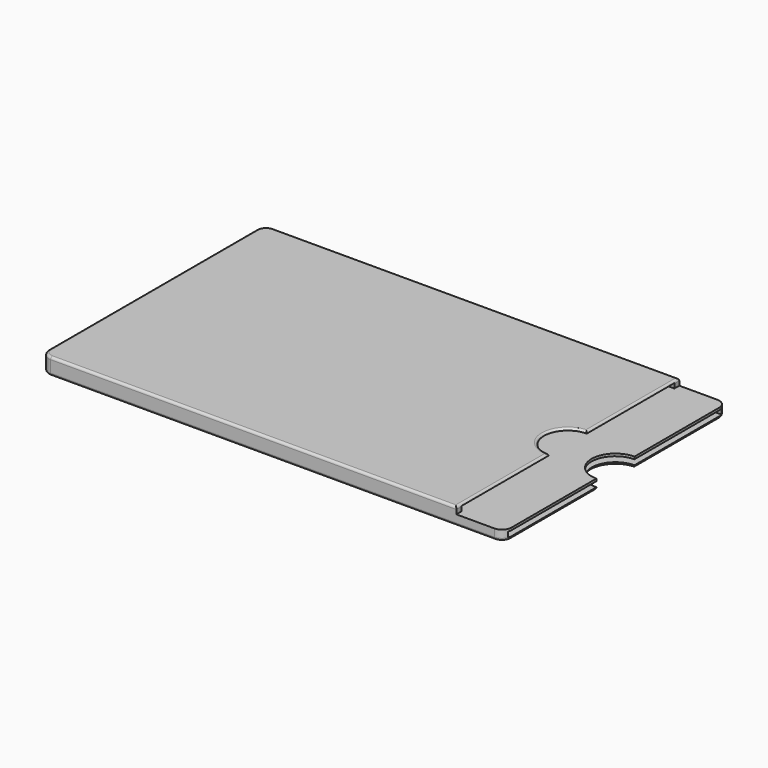
from build123d import *

# Parameters (mm, degrees)
F0_W         = 10
F0_H         = 56
F1_DEPTH     = 3
F2_DEPTH     = 2.6
F4_DEPTH     = 1.6
F5_DEPTH     = 1.1
F6_DEPTH     = 0.5
F7_T1_DEPTH  = 13.5
F7_T3_DEPTH  = 12.1
F8_T1_DEPTH  = 86.55
F8_T3_DEPTH  = 54.6
F8_T5_DEPTH  = 26.8
F8_T7_DEPTH  = 26.8
F8_T9_DEPTH  = 93.3
F8_T11_DEPTH = 23.55
F8_T13_DEPTH = 23.55
F8_T16_ANGLE = 89.9999999857
F8_T18_ANGLE = 208.1142252403
F8_T20_ANGLE = 89.9999999955
F8_T22_ANGLE = 89.9999999857
F8_T24_ANGLE = 89.9999999955
F8_T26_ANGLE = 208.6939609801
F8_T28_ANGLE = 90.0000000053
F8_T30_ANGLE = 89.9999999955


# Not quite as in the source:
# - a fillet or chamfer that OpenCascade refuses, or shapes differently, is made with other operations: its cross-section is extruded or revolved along the edge and cut away or added


with BuildPart() as f1:
    # F0 (on Top) → F1 (new body)
    with BuildSketch(Plane.XY):
        Polygon((-58.3780704141, -12.1535575017), (-58.3780704141, 43.8464424983), (-48.3780704141, 43.8464424983), (27.6219295859, 43.8464424983), (27.6219295859, 45.1464424983), (-59.6780704141, 45.1464424983), (-59.6780704141, -13.4535575017), (27.6219295859, -13.4535575017), (27.6219295859, -12.1535575017), (-48.3780704141, -12.1535575017), align=None)
        with Locations((-53.3780704141, 15.8464424983)):
            Rectangle(F0_W, F0_H)
        with BuildLine():
            Line((27.6219295859, 43.8464424983), (-48.3780704141, 43.8464424983))
            Line((-48.3780704141, 43.8464424983), (-48.3780704141, -12.1535575017))
            Line((-48.3780704141, -12.1535575017), (27.6219295859, -12.1535575017))
            Line((27.6219295859, -12.1535575017), (27.6219295859, 10.8464424983))
            ThreePointArc((27.6219295859, 10.8464424983), (22.6219295859, 15.8464424983), (27.6219295859, 20.8464424983))
            Line((27.6219295859, 20.8464424983), (27.6219295859, 43.8464424983))
        make_face()
    extrude(amount=F1_DEPTH)

    # F0 (on Top) → F2 (cut)
    with BuildSketch(Plane.XY):
        with Locations((-53.3780704141, 15.8464424983)):
            Rectangle(F0_W, F0_H)
        with BuildLine():
            Line((27.6219295859, 43.8464424983), (-48.3780704141, 43.8464424983))
            Line((-48.3780704141, 43.8464424983), (-48.3780704141, -12.1535575017))
            Line((-48.3780704141, -12.1535575017), (27.6219295859, -12.1535575017))
            Line((27.6219295859, -12.1535575017), (27.6219295859, 10.8464424983))
            ThreePointArc((27.6219295859, 10.8464424983), (22.6219295859, 15.8464424983), (27.6219295859, 20.8464424983))
            Line((27.6219295859, 20.8464424983), (27.6219295859, 43.8464424983))
        make_face()
    extrude(amount=F2_DEPTH, mode=Mode.SUBTRACT)

    # F0 (on Top) + F3 (on Top) → F4 (join)
    with BuildSketch(Plane.XY):
        with BuildLine():
            Line((27.6219295859, 43.8464424983), (-48.3780704141, 43.8464424983))
            Line((-48.3780704141, 43.8464424983), (-48.3780704141, -12.1535575017))
            Line((-48.3780704141, -12.1535575017), (27.6219295859, -12.1535575017))
            Line((27.6219295859, -12.1535575017), (27.6219295859, 10.8464424983))
            ThreePointArc((27.6219295859, 10.8464424983), (22.6219295859, 15.8464424983), (27.6219295859, 20.8464424983))
            Line((27.6219295859, 20.8464424983), (27.6219295859, 43.8464424983))
        make_face()
        with BuildLine():
            Line((27.6219295859, 10.8464424983), (27.6219295859, 20.8464424983))
            ThreePointArc((27.6219295859, 20.8464424983), (22.6219295859, 15.8464424983), (27.6219295859, 10.8464424983))
        make_face()
        with Locations((-53.3780704141, 15.8464424983)):
            Rectangle(F0_W, F0_H)
    with BuildSketch(Plane.XY):
        with BuildLine():
            Line((37.6219295859, 20.8464424983), (37.6219295859, 45.1464424983))
            Line((37.6219295859, 45.1464424983), (27.6219295859, 45.1464424983))
            Line((27.6219295859, 45.1464424983), (27.6219295859, -13.4535575017))
            Line((27.6219295859, -13.4535575017), (37.6219295859, -13.4535575017))
            Line((37.6219295859, -13.4535575017), (37.6219295859, 10.8464424983))
            ThreePointArc((37.6219295859, 10.8464424983), (32.6219295859, 15.8464424983), (37.6219295859, 20.8464424983))
        make_face()
    extrude(amount=F4_DEPTH)

    # F0 (on Top) → F5 (cut)
    with BuildSketch(Plane.XY):
        Polygon((37.6219295859, 43.8464424983), (27.6219295859, 43.8464424983), (27.6219295859, 20.8464424983), (27.6219295859, 10.8464424983), (27.6219295859, -12.1535575017), (37.6219295859, -12.1535575017), align=None)
        with BuildLine():
            Line((27.6219295859, 43.8464424983), (-48.3780704141, 43.8464424983))
            Line((-48.3780704141, 43.8464424983), (-48.3780704141, -12.1535575017))
            Line((-48.3780704141, -12.1535575017), (27.6219295859, -12.1535575017))
            Line((27.6219295859, -12.1535575017), (27.6219295859, 10.8464424983))
            ThreePointArc((27.6219295859, 10.8464424983), (22.6219295859, 15.8464424983), (27.6219295859, 20.8464424983))
            Line((27.6219295859, 20.8464424983), (27.6219295859, 43.8464424983))
        make_face()
        with BuildLine():
            Line((27.6219295859, 10.8464424983), (27.6219295859, 20.8464424983))
            ThreePointArc((27.6219295859, 20.8464424983), (22.6219295859, 15.8464424983), (27.6219295859, 10.8464424983))
        make_face()
    extrude(amount=F5_DEPTH, mode=Mode.SUBTRACT)

    # F0 (on Top) + F3 (on Top) → F6 (join)
    with BuildSketch(Plane.XY):
        with BuildLine():
            Line((27.6219295859, 43.8464424983), (-48.3780704141, 43.8464424983))
            Line((-48.3780704141, 43.8464424983), (-48.3780704141, -12.1535575017))
            Line((-48.3780704141, -12.1535575017), (27.6219295859, -12.1535575017))
            Line((27.6219295859, -12.1535575017), (27.6219295859, 10.8464424983))
            ThreePointArc((27.6219295859, 10.8464424983), (22.6219295859, 15.8464424983), (27.6219295859, 20.8464424983))
            Line((27.6219295859, 20.8464424983), (27.6219295859, 43.8464424983))
        make_face()
        with BuildLine():
            Line((27.6219295859, 10.8464424983), (27.6219295859, 20.8464424983))
            ThreePointArc((27.6219295859, 20.8464424983), (22.6219295859, 15.8464424983), (27.6219295859, 10.8464424983))
        make_face()
        with Locations((-53.3780704141, 15.8464424983)):
            Rectangle(F0_W, F0_H)
        Polygon((-58.3780704141, -12.1535575017), (-58.3780704141, 43.8464424983), (-48.3780704141, 43.8464424983), (27.6219295859, 43.8464424983), (27.6219295859, 45.1464424983), (-59.6780704141, 45.1464424983), (-59.6780704141, -13.4535575017), (27.6219295859, -13.4535575017), (27.6219295859, -12.1535575017), (-48.3780704141, -12.1535575017), align=None)
    with BuildSketch(Plane.XY):
        with BuildLine():
            Line((37.6219295859, 20.8464424983), (37.6219295859, 45.1464424983))
            Line((37.6219295859, 45.1464424983), (27.6219295859, 45.1464424983))
            Line((27.6219295859, 45.1464424983), (27.6219295859, -13.4535575017))
            Line((27.6219295859, -13.4535575017), (37.6219295859, -13.4535575017))
            Line((37.6219295859, -13.4535575017), (37.6219295859, 10.8464424983))
            ThreePointArc((37.6219295859, 10.8464424983), (32.6219295859, 15.8464424983), (37.6219295859, 20.8464424983))
        make_face()
    extrude(amount=-F6_DEPTH)

    # F7: fillet of radius 2 on 4 edges, made by hand

    # F7_s2 → F7_t1 (cut)
    with BuildSketch(Plane.XY.offset(-5.5)):
        with BuildLine():
            ThreePointArc((-57.6780704141, 45.1464424983), (-59.0922839764, 44.5606560606), (-59.6780704141, 43.1464424983))
            Line((-59.6780704141, 43.1464424983), (-59.6780704141, 45.1464424983))
            Line((-59.6780704141, 45.1464424983), (-57.6780704141, 45.1464424983))
        make_face()
        with BuildLine():
            ThreePointArc((-57.6780704141, -13.4535575017), (-59.0922839764, -12.8677710641), (-59.6780704141, -11.4535575017))
            Line((-59.6780704141, -11.4535575017), (-59.6780704141, -13.4535575017))
            Line((-59.6780704141, -13.4535575017), (-57.6780704141, -13.4535575017))
        make_face()
    extrude(amount=F7_T1_DEPTH, mode=Mode.SUBTRACT)

    # F7_s4 → F7_t3 (cut)
    with BuildSketch(Plane.XY.offset(-5.5)):
        with BuildLine():
            ThreePointArc((37.6219295859, -11.4535575017), (37.0361431483, -12.8677710641), (35.6219295859, -13.4535575017))
            Line((35.6219295859, -13.4535575017), (37.6219295859, -13.4535575017))
            Line((37.6219295859, -13.4535575017), (37.6219295859, -11.4535575017))
        make_face()
        with BuildLine():
            ThreePointArc((35.6219295859, 45.1464424983), (37.0361431483, 44.5606560606), (37.6219295859, 43.1464424983))
            Line((37.6219295859, 43.1464424983), (37.6219295859, 45.1464424983))
            Line((37.6219295859, 45.1464424983), (35.6219295859, 45.1464424983))
        make_face()
    extrude(amount=F7_T3_DEPTH, mode=Mode.SUBTRACT)

    # F8: fillet of radius 0.5 on 18 edges, made by hand

    # F8_s2 → F8_t1 (cut)
    with BuildSketch(Plane.YZ.offset(-57.6780704141)):
        with BuildLine():
            ThreePointArc((45.1464424983, 2.5), (44.9999958889, 2.8535533906), (44.6464424983, 3))
            Line((44.6464424983, 3), (45.1464424983, 3))
            Line((45.1464424983, 3), (45.1464424983, 2.5))
        make_face()
        with BuildLine():
            ThreePointArc((-12.9535575017, 3), (-13.3071108923, 2.8535533906), (-13.4535575017, 2.5))
            Line((-13.4535575017, 2.5), (-13.4535575017, 3))
            Line((-13.4535575017, 3), (-12.9535575017, 3))
        make_face()
    extrude(amount=F8_T1_DEPTH, mode=Mode.SUBTRACT)

    # F8_s4 → F8_t3 (cut)
    with BuildSketch(Plane.XZ.offset(-43.1464424983)):
        with BuildLine():
            ThreePointArc((-59.1780704141, 3), (-59.5316238047, 2.8535533906), (-59.6780704141, 2.5))
            Line((-59.6780704141, 2.5), (-59.6780704141, 3))
            Line((-59.6780704141, 3), (-59.1780704141, 3))
        make_face()
        with BuildLine():
            ThreePointArc((-59.1780704141, -0.5), (-59.5316238047, -0.3535533906), (-59.6780704141, 0))
            Line((-59.6780704141, 0), (-59.6780704141, -0.5))
            Line((-59.6780704141, -0.5), (-59.1780704141, -0.5))
        make_face()
    extrude(amount=F8_T3_DEPTH, mode=Mode.SUBTRACT)

    # F8_s6 → F8_t5 (cut)
    with BuildSketch(Plane.XZ.offset(-46.3964424983)):
        with BuildLine():
            ThreePointArc((27.1219295859, 3), (27.4754829765, 2.8535533906), (27.6219295859, 2.5))
            Line((27.6219295859, 2.5), (27.6219295859, 3))
            Line((27.6219295859, 3), (27.1219295859, 3))
        make_face()
    extrude(amount=F8_T5_DEPTH, mode=Mode.SUBTRACT)

    # F8_s8 → F8_t7 (cut)
    with BuildSketch(Plane.XZ.offset(-12.0964424983)):
        with BuildLine():
            ThreePointArc((27.1219295859, 3), (27.4754829765, 2.8535533906), (27.6219295859, 2.5))
            Line((27.6219295859, 2.5), (27.6219295859, 3))
            Line((27.6219295859, 3), (27.1219295859, 3))
        make_face()
    extrude(amount=F8_T7_DEPTH, mode=Mode.SUBTRACT)

    # F8_s10 → F8_t9 (cut)
    with BuildSketch(Plane.YZ.offset(-57.6780704141)):
        with BuildLine():
            ThreePointArc((45.1464424983, 0), (44.9999958889, -0.3535533906), (44.6464424983, -0.5))
            Line((44.6464424983, -0.5), (45.1464424983, -0.5))
            Line((45.1464424983, -0.5), (45.1464424983, 0))
        make_face()
        with BuildLine():
            ThreePointArc((-12.9535575017, -0.5), (-13.3071108923, -0.3535533906), (-13.4535575017, 0))
            Line((-13.4535575017, 0), (-13.4535575017, -0.5))
            Line((-13.4535575017, -0.5), (-12.9535575017, -0.5))
        make_face()
    extrude(amount=F8_T9_DEPTH, mode=Mode.SUBTRACT)

    # F8_s12 → F8_t11 (cut)
    with BuildSketch(Plane.XZ.offset(-43.1464424983)):
        with BuildLine():
            ThreePointArc((37.1219295859, -0.5), (37.4754829765, -0.3535533906), (37.6219295859, 0))
            Line((37.6219295859, 0), (37.6219295859, -0.5))
            Line((37.6219295859, -0.5), (37.1219295859, -0.5))
        make_face()
    extrude(amount=F8_T11_DEPTH, mode=Mode.SUBTRACT)

    # F8_s14 → F8_t13 (cut)
    with BuildSketch(Plane.XZ.offset(-12.0964424983)):
        with BuildLine():
            ThreePointArc((37.1219295859, -0.5), (37.4754829765, -0.3535533906), (37.6219295859, 0))
            Line((37.6219295859, 0), (37.6219295859, -0.5))
            Line((37.6219295859, -0.5), (37.1219295859, -0.5))
        make_face()
    extrude(amount=F8_T13_DEPTH, mode=Mode.SUBTRACT)

    # F8_s15 → F8_t16 (revolve, cut)
    with BuildSketch(Plane.XZ.offset(-43.1464424981)):
        with BuildLine():
            ThreePointArc((-59.6780704141, 2.5), (-59.5316238047, 2.8535533906), (-59.1780704141, 3))
            Line((-59.1780704141, 3), (-59.6780704141, 3))
            Line((-59.6780704141, 3), (-59.6780704141, 2.5))
        make_face()
    revolve(axis=Axis((-57.6780704139, 43.1464424981, 3), (0, 0, -1)), revolution_arc=F8_T16_ANGLE, mode=Mode.SUBTRACT)

    # F8_s17 → F8_t18 (revolve, cut)
    with BuildSketch(Plane(origin=(29.7260389432, 7.4430147649, 0), x_dir=(0, 0, 1), z_dir=(0.9700540957, 0.2428889692, 0))):
        with BuildLine():
            ThreePointArc((3, -3.1729464952), (2.8872983346, -3.4891742612), (2.6, -3.6628444437))
            Line((2.6, -3.6628444437), (3, -3.6628444437))
            Line((3, -3.6628444437), (3, -3.1729464952))
        make_face()
    revolve(axis=Axis((27.6219295859, 15.8464424983, 3), (0, 0, -1)), revolution_arc=F8_T18_ANGLE, mode=Mode.SUBTRACT)

    # F8_s19 → F8_t20 (revolve, cut)
    with BuildSketch(Plane.YZ.offset(-57.678070414)):
        with BuildLine():
            ThreePointArc((-12.9535575017, 3), (-13.3071108923, 2.8535533906), (-13.4535575017, 2.5))
            Line((-13.4535575017, 2.5), (-13.4535575017, 3))
            Line((-13.4535575017, 3), (-12.9535575017, 3))
        make_face()
    revolve(axis=Axis((-57.678070414, -11.4535575016, 3), (0, 0, -1)), revolution_arc=F8_T20_ANGLE, mode=Mode.SUBTRACT)

    # F8_s21 → F8_t22 (revolve, cut)
    with BuildSketch(Plane.XZ.offset(-43.1464424981)):
        with BuildLine():
            ThreePointArc((-59.1780704141, -0.5), (-59.5316238047, -0.3535533906), (-59.6780704141, 0))
            Line((-59.6780704141, 0), (-59.6780704141, -0.5))
            Line((-59.6780704141, -0.5), (-59.1780704141, -0.5))
        make_face()
    revolve(axis=Axis((-57.6780704139, 43.1464424981, -0.5), (0, 0, -1)), revolution_arc=F8_T22_ANGLE, mode=Mode.SUBTRACT)

    # F8_s23 → F8_t24 (revolve, cut)
    with BuildSketch(Plane.YZ.offset(35.6219295858)):
        with BuildLine():
            ThreePointArc((45.1464424983, 0), (44.9999958889, -0.3535533906), (44.6464424983, -0.5))
            Line((44.6464424983, -0.5), (45.1464424983, -0.5))
            Line((45.1464424983, -0.5), (45.1464424983, 0))
        make_face()
    revolve(axis=Axis((35.6219295858, 43.1464424982, -0.5), (0, 0, -1)), revolution_arc=F8_T24_ANGLE, mode=Mode.SUBTRACT)

    # F8_s25 → F8_t26 (revolve, cut)
    with BuildSketch(Plane(origin=(39.1160669209, 10.0047252674, 0), x_dir=(0, 0, 1), z_dir=(0.9688128753, 0.2477934878, 0))):
        with BuildLine():
            ThreePointArc((-0.5, -0.5297683688), (-0.3535533906, -0.8833217594), (0, -1.0297683688))
            Line((0, -1.0297683688), (-0.5, -1.0297683688))
            Line((-0.5, -1.0297683688), (-0.5, -0.5297683688))
        make_face()
    revolve(axis=Axis((37.6219295859, 15.8464424983, -0.5), (0, 0, -1)), revolution_arc=F8_T26_ANGLE, mode=Mode.SUBTRACT)

    # F8_s27 → F8_t28 (revolve, cut)
    with BuildSketch(Plane.XZ.offset(11.4535575018)):
        with BuildLine():
            ThreePointArc((37.1219295859, -0.5), (37.4754829765, -0.3535533906), (37.6219295859, 0))
            Line((37.6219295859, 0), (37.6219295859, -0.5))
            Line((37.6219295859, -0.5), (37.1219295859, -0.5))
        make_face()
    revolve(axis=Axis((35.621929586, -11.4535575018, -0.5), (0, 0, -1)), revolution_arc=F8_T28_ANGLE, mode=Mode.SUBTRACT)

    # F8_s29 → F8_t30 (revolve, cut)
    with BuildSketch(Plane.YZ.offset(-57.678070414)):
        with BuildLine():
            ThreePointArc((-12.9535575017, -0.5), (-13.3071108923, -0.3535533906), (-13.4535575017, 0))
            Line((-13.4535575017, 0), (-13.4535575017, -0.5))
            Line((-13.4535575017, -0.5), (-12.9535575017, -0.5))
        make_face()
    revolve(axis=Axis((-57.678070414, -11.4535575016, -0.5), (0, 0, -1)), revolution_arc=F8_T30_ANGLE, mode=Mode.SUBTRACT)


solid = f1.part
